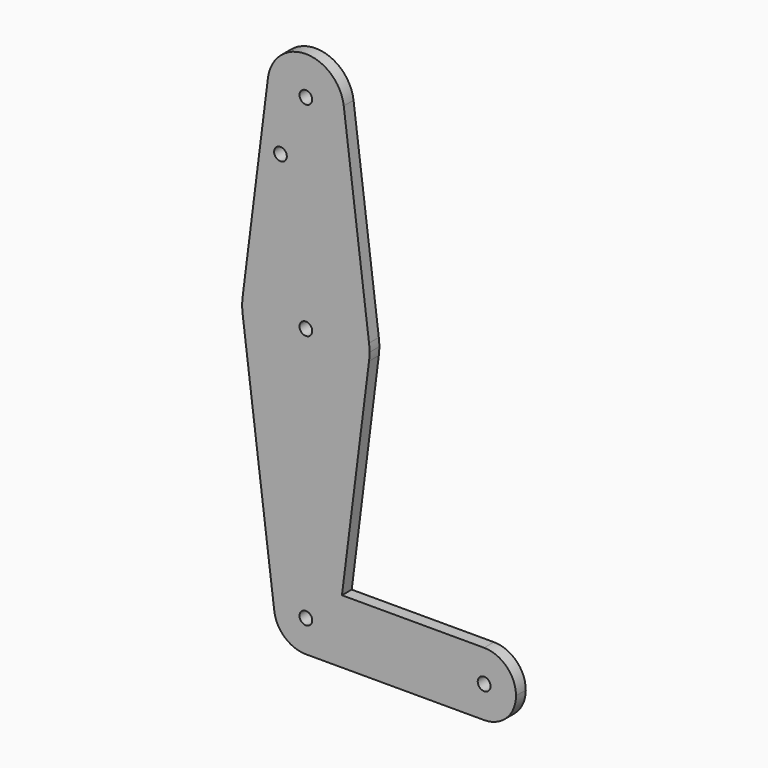
from build123d import *

# Parameters (mm, degrees)
F0_R     = 1.5875
F0_R_2   = 1.6002
F1_DEPTH = 3.048
F4_DEPTH = 3.048


# Not quite as in the source:
# - a feature of the source that left no trace in its solid (it failed there, or was rolled back) is left out


with BuildPart() as f1:
    # F0 (on Front) → F1 (new body)
    with BuildSketch(Plane.XZ):
        with BuildLine():
            ThreePointArc((-9.4502929642, 115.490625), (-0.596483242, 104.7936951058), (9.525, 114.3))
            ThreePointArc((9.525, 114.3), (9.5063048942, 114.896483242), (9.4502929642, 115.490625))
            ThreePointArc((9.4502929642, 115.490625), (0, 123.825), (-9.4502929642, 115.490625))
        make_face()
        with Locations((0, 114.3)):
            Circle(F0_R, mode=Mode.SUBTRACT)
        with BuildLine():
            ThreePointArc((9.4502929642, 115.490625), (9.5063048942, 114.896483242), (9.525, 114.3))
            ThreePointArc((9.525, 114.3), (-0.596483242, 104.7936951058), (-9.4502929642, 115.490625))
            Line((-9.4502929642, 115.490625), (-15.7504882737, 65.484375))
            ThreePointArc((-15.7504882737, 65.484375), (0, 79.375), (15.7504882737, 65.484375))
            Line((15.7504882737, 65.484375), (9.4502929642, 115.490625))
        make_face()
        with Locations((-6.3295518048, 99.7836068273)):
            Circle(F0_R, mode=Mode.SUBTRACT)
        with BuildLine():
            ThreePointArc((15.875, 63.5), (15.8438414904, 64.4941387366), (15.7504882737, 65.484375))
            ThreePointArc((15.7504882737, 65.484375), (0, 79.375), (-15.7504882737, 65.484375))
            ThreePointArc((-15.7504882737, 65.484375), (-15.875, 63.5), (-15.7504882737, 61.515625))
            ThreePointArc((-15.7504882737, 61.515625), (0, 47.625), (15.7504882737, 61.515625))
            ThreePointArc((15.7504882737, 61.515625), (15.8438414904, 62.5058612634), (15.875, 63.5))
        make_face()
        with Locations((0, 63.5)):
            Circle(F0_R, mode=Mode.SUBTRACT)
        with BuildLine():
            ThreePointArc((15.7504882737, 61.515625), (0, 47.625), (-15.7504882737, 61.515625))
            Line((-15.7504882737, 61.515625), (-7.8752441368, -0.9921875))
            ThreePointArc((-7.8752441368, -0.9921875), (-5.953125, 5.2501627579), (0, 7.9375))
            Line((0, 7.9375), (9.0002790135, 7.9375))
            Line((9.0002790135, 7.9375), (15.7504882737, 61.515625))
        make_face()
        with BuildLine():
            ThreePointArc((0, 7.9375), (-5.953125, 5.2501627579), (-7.8752441368, -0.9921875))
            ThreePointArc((-7.8752441368, -0.9921875), (-5.2501627579, -5.953125), (0, -7.9375))
            ThreePointArc((0, -7.9375), (5.2501627579, -5.953125), (7.8752441368, -0.9921875))
            ThreePointArc((7.8752441368, -0.9921875), (7.9219207452, -0.4970693683), (7.9375, 0))
            ThreePointArc((7.9375, 0), (5.6126600757, 5.6126600757), (0, 7.9375))
        make_face()
        Circle(F0_R, mode=Mode.SUBTRACT)
        with BuildLine():
            Line((7.8752441368, -0.9921875), (9.0002790135, 7.9375))
            Line((9.0002790135, 7.9375), (0, 7.9375))
            ThreePointArc((0, 7.9375), (5.6126600757, 5.6126600757), (7.9375, 0))
            ThreePointArc((7.9375, 0), (7.9219207452, -0.4970693683), (7.8752441368, -0.9921875))
        make_face()
        with BuildLine():
            Line((44.45, 7.9375), (9.0002790135, 7.9375))
            Line((9.0002790135, 7.9375), (7.8752441368, -0.9921875))
            ThreePointArc((7.8752441368, -0.9921875), (5.2501627579, -5.953125), (0, -7.9375))
            Line((0, -7.9375), (44.45, -7.9375))
            ThreePointArc((44.45, -7.9375), (36.5125, 0), (44.45, 7.9375))
        make_face()
        with BuildLine():
            ThreePointArc((52.3875, 0), (50.0626600757, 5.6126600757), (44.45, 7.9375))
            ThreePointArc((44.45, 7.9375), (36.5125, 0), (44.45, -7.9375))
            ThreePointArc((44.45, -7.9375), (50.0626600757, -5.6126600757), (52.3875, 0))
        make_face()
        with Locations((44.45, 0)):
            Circle(F0_R_2, mode=Mode.SUBTRACT)
    extrude(amount=F1_DEPTH)


with BuildPart() as f4:
    # F0 (on Front) → F4 (new body)
    with BuildSketch(Plane.XZ):
        with BuildLine():
            ThreePointArc((-9.4502929642, 115.490625), (-0.596483242, 104.7936951058), (9.525, 114.3))
            ThreePointArc((9.525, 114.3), (9.5063048942, 114.896483242), (9.4502929642, 115.490625))
            ThreePointArc((9.4502929642, 115.490625), (0, 123.825), (-9.4502929642, 115.490625))
        make_face()
        with Locations((0, 114.3)):
            Circle(F0_R, mode=Mode.SUBTRACT)
        with BuildLine():
            ThreePointArc((9.4502929642, 115.490625), (9.5063048942, 114.896483242), (9.525, 114.3))
            ThreePointArc((9.525, 114.3), (-0.596483242, 104.7936951058), (-9.4502929642, 115.490625))
            Line((-9.4502929642, 115.490625), (-15.7504882737, 65.484375))
            ThreePointArc((-15.7504882737, 65.484375), (0, 79.375), (15.7504882737, 65.484375))
            Line((15.7504882737, 65.484375), (9.4502929642, 115.490625))
        make_face()
        with Locations((-6.3295518048, 99.7836068273)):
            Circle(F0_R, mode=Mode.SUBTRACT)
        with BuildLine():
            ThreePointArc((15.875, 63.5), (15.8438414904, 64.4941387366), (15.7504882737, 65.484375))
            ThreePointArc((15.7504882737, 65.484375), (0, 79.375), (-15.7504882737, 65.484375))
            ThreePointArc((-15.7504882737, 65.484375), (-15.875, 63.5), (-15.7504882737, 61.515625))
            ThreePointArc((-15.7504882737, 61.515625), (0, 47.625), (15.7504882737, 61.515625))
            ThreePointArc((15.7504882737, 61.515625), (15.8438414904, 62.5058612634), (15.875, 63.5))
        make_face()
        with Locations((0, 63.5)):
            Circle(F0_R, mode=Mode.SUBTRACT)
        with BuildLine():
            ThreePointArc((15.7504882737, 61.515625), (0, 47.625), (-15.7504882737, 61.515625))
            Line((-15.7504882737, 61.515625), (-7.8752441368, -0.9921875))
            ThreePointArc((-7.8752441368, -0.9921875), (-5.953125, 5.2501627579), (0, 7.9375))
            Line((0, 7.9375), (9.0002790135, 7.9375))
            Line((9.0002790135, 7.9375), (15.7504882737, 61.515625))
        make_face()
        with BuildLine():
            ThreePointArc((0, 7.9375), (-5.953125, 5.2501627579), (-7.8752441368, -0.9921875))
            ThreePointArc((-7.8752441368, -0.9921875), (-5.2501627579, -5.953125), (0, -7.9375))
            ThreePointArc((0, -7.9375), (5.2501627579, -5.953125), (7.8752441368, -0.9921875))
            ThreePointArc((7.8752441368, -0.9921875), (7.9219207452, -0.4970693683), (7.9375, 0))
            ThreePointArc((7.9375, 0), (5.6126600757, 5.6126600757), (0, 7.9375))
        make_face()
        Circle(F0_R, mode=Mode.SUBTRACT)
        with BuildLine():
            Line((7.8752441368, -0.9921875), (9.0002790135, 7.9375))
            Line((9.0002790135, 7.9375), (0, 7.9375))
            ThreePointArc((0, 7.9375), (5.6126600757, 5.6126600757), (7.9375, 0))
            ThreePointArc((7.9375, 0), (7.9219207452, -0.4970693683), (7.8752441368, -0.9921875))
        make_face()
        with BuildLine():
            Line((44.45, 7.9375), (9.0002790135, 7.9375))
            Line((9.0002790135, 7.9375), (7.8752441368, -0.9921875))
            ThreePointArc((7.8752441368, -0.9921875), (5.2501627579, -5.953125), (0, -7.9375))
            Line((0, -7.9375), (44.45, -7.9375))
            ThreePointArc((44.45, -7.9375), (36.5125, 0), (44.45, 7.9375))
        make_face()
        with BuildLine():
            ThreePointArc((52.3875, 0), (50.0626600757, 5.6126600757), (44.45, 7.9375))
            ThreePointArc((44.45, 7.9375), (36.5125, 0), (44.45, -7.9375))
            ThreePointArc((44.45, -7.9375), (50.0626600757, -5.6126600757), (52.3875, 0))
        make_face()
        with Locations((44.45, 0)):
            Circle(F0_R_2, mode=Mode.SUBTRACT)
    extrude(amount=F4_DEPTH)


solid = f4.part
